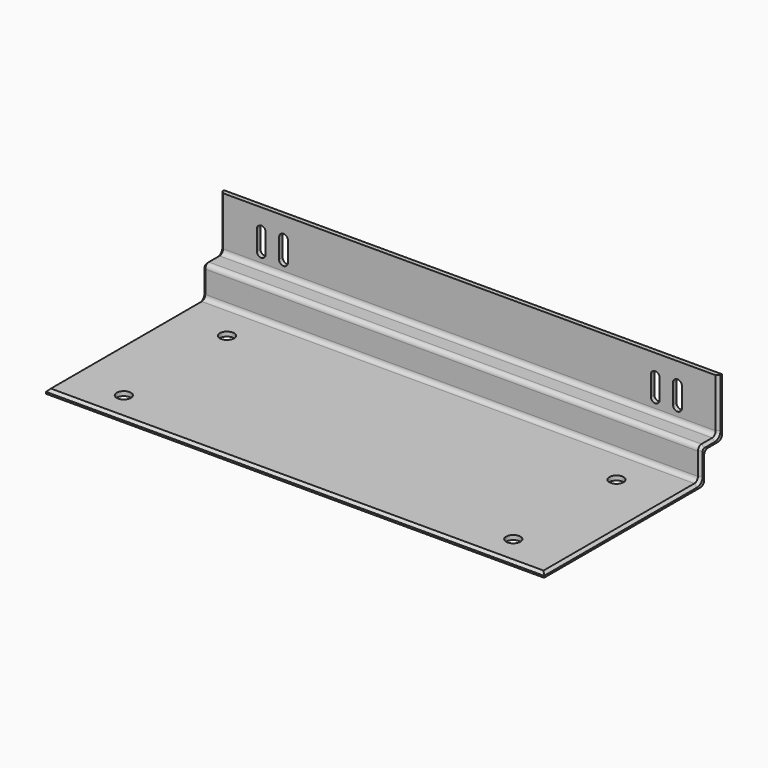
from build123d import *

# Parameters (mm, degrees)
F1_DEPTH     = 560
F3_DEPTH     = 5.001
F5_SIZE      = 3
F6_SIZE      = 3
F7_SIZE      = 3
F4_R         = 8
F8_DEPTH     = 25
F9_TEXT_SIZE = 17.1886394835
F10_DEPTH    = 1.5


# Not quite as in the source:
# - Text() gives the source's letters only with a copy of the font that has no kerning and outlines rounded to 1/6400 em; it was checked with that copy


with BuildPart() as f1:
    # F0 (on Right) → F1 (new body)
    with BuildSketch(Plane.YZ):
        with BuildLine():
            Line((0, -60), (0, 0))
            Line((0, 0), (-5, 0))
            Line((-5, 0), (-5, -55))
            ThreePointArc((-5, -55), (-6.4644660941, -58.5355339059), (-10, -60))
            Line((-10, -60), (-25, -60))
            ThreePointArc((-25, -60), (-28.5355339059, -61.4644660941), (-30, -65))
            Line((-30, -65), (-30, -90))
            ThreePointArc((-30, -90), (-31.4644660941, -93.5355339059), (-35, -95))
            Line((-35, -95), (-250, -95))
            Line((-250, -95), (-250, -100))
            Line((-250, -100), (-30, -100))
            ThreePointArc((-30, -100), (-26.4644660941, -98.5355339059), (-25, -95))
            Line((-25, -95), (-25, -70))
            ThreePointArc((-25, -70), (-23.5355339059, -66.4644660941), (-20, -65))
            Line((-20, -65), (-5, -65))
            ThreePointArc((-5, -65), (-1.4644660941, -63.5355339059), (0, -60))
        make_face()
    extrude(amount=F1_DEPTH)

    # F2 (on face) → F3 (cut, through all)
    with BuildSketch(Plane.XZ.offset(5)):
        with BuildLine():
            Line((494, -45), (494, -23))
            ThreePointArc((494, -23), (492.5355339059, -19.4644660941), (489, -18))
            ThreePointArc((489, -18), (485.4644660941, -19.4644660941), (484, -23))
            Line((484, -23), (484, -45))
            ThreePointArc((484, -45), (485.4644670927, -48.5355349046), (489.0000028246, -50))
            ThreePointArc((489.0000028246, -50), (492.5355349046, -48.5355329073), (494, -45))
        make_face()
        with BuildLine():
            Line((519, -45), (519, -23))
            ThreePointArc((519, -23), (517.5355339059, -19.4644660941), (514, -18))
            ThreePointArc((514, -18), (510.4644660941, -19.4644660941), (509, -23))
            Line((509, -23), (509, -45))
            ThreePointArc((509, -45), (510.4644670927, -48.5355349046), (514.0000028246, -50))
            ThreePointArc((514.0000028246, -50), (517.5355349046, -48.5355329073), (519, -45))
        make_face()
        with BuildLine():
            ThreePointArc((45.9999971754, -50), (49.5355329073, -48.5355349046), (51, -45))
            Line((51, -45), (51, -23))
            ThreePointArc((51, -23), (49.5355339059, -19.4644660941), (46, -18))
            ThreePointArc((46, -18), (42.4644660941, -19.4644660941), (41, -23))
            Line((41, -23), (41, -45))
            ThreePointArc((41, -45), (42.4644650954, -48.5355329073), (45.9999971754, -50))
        make_face()
        with BuildLine():
            ThreePointArc((66, -45), (67.4644650954, -48.5355329073), (70.9999971754, -50))
            ThreePointArc((70.9999971754, -50), (74.5355329073, -48.5355349046), (76, -45))
            Line((76, -45), (76, -23))
            ThreePointArc((76, -23), (74.5355339059, -19.4644660941), (71, -18))
            ThreePointArc((71, -18), (67.4644660941, -19.4644660941), (66, -23))
            Line((66, -23), (66, -45))
        make_face()
    extrude(amount=-F3_DEPTH, mode=Mode.SUBTRACT)

    # F5
    f5_edges = [f1.edges().sort_by_distance(p)[0] for p in [
        (280, -250, -95),
    ]]
    chamfer(f5_edges, length=F5_SIZE)

    # F6
    f6_edges = [f1.edges().sort_by_distance(p)[0] for p in [
        (0, -141, -95),
    ]]
    chamfer(f6_edges, length=F6_SIZE)

    # F7
    f7_edges = [f1.edges().sort_by_distance(p)[0] for p in [
        (560, -141, -95),
    ]]
    chamfer(f7_edges, length=F7_SIZE)

    # F4 (on face) → F8 (cut)
    with BuildSketch(Plane.XY.offset(-95)):
        with Locations((61, -217)):
            Circle(F4_R)
        with Locations((499, -217)):
            Circle(F4_R)
        with Locations((61, -72)):
            Circle(F4_R)
        with Locations((499, -72)):
            Circle(F4_R)
    extrude(amount=-F8_DEPTH, mode=Mode.SUBTRACT)

    # F9 (on face) → F10 (cut)
    with BuildSketch(Plane(origin=(0, 0, -100), x_dir=(1, 0, 0), z_dir=(0, 0, -1))):
        with Locations((407.9401791096, 37.7891585231)):
            Text('Regalboden 56 cm', F9_TEXT_SIZE, font='Open Sans', text_align=(TextAlign.LEFT, TextAlign.BOTTOM))
    extrude(amount=-F10_DEPTH, mode=Mode.SUBTRACT)


solid = f1.part
